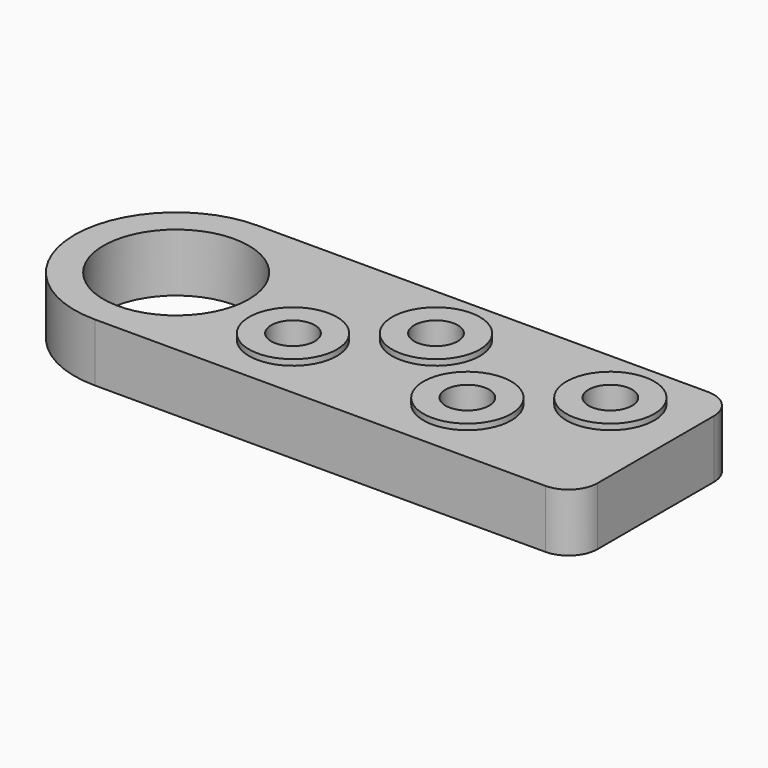
from build123d import *

# Parameters (mm, degrees)
F0_R         = 12.5
F1_DEPTH     = 10
F2_R         = 7.55
F2_R_2       = 3.75
F3_DEPTH     = 1
F4_DEPTH     = 9
F5_TEXT_SIZE = 5.5555555556
F6_DEPTH     = 1


# Not quite as in the source:
# - Text() gives the source's letters only with a copy of the font that has no kerning and outlines rounded to 1/6400 em; it was checked with that copy


with BuildPart() as f1:
    # F0 (on Top) → F1 (new body)
    with BuildSketch(Plane.XY):
        with BuildLine():
            ThreePointArc((0, 17.5), (5.1256313292, 5.1256313292), (17.5, 0))
            Line((17.5, 0), (95, 0))
            ThreePointArc((95, 0), (98.5355339059, 1.4644660941), (100, 5))
            Line((100, 5), (100, 30))
            ThreePointArc((100, 30), (98.5355339059, 33.5355339059), (95, 35))
            Line((95, 35), (17.5, 35))
            ThreePointArc((17.5, 35), (5.1256313292, 29.8743686708), (0, 17.5))
        make_face()
        with Locations((17.5, 17.5)):
            Circle(F0_R, mode=Mode.SUBTRACT)
    extrude(amount=F1_DEPTH)

    # F2 (on face) → F3 (join)
    with BuildSketch(Plane.XY.offset(10)):
        with Locations((42, 12)):
            Circle(F2_R)
        with Locations((42, 12)):
            Circle(F2_R_2, mode=Mode.SUBTRACT)
        with Locations((57, 24)):
            Circle(F2_R)
        with Locations((57, 24)):
            Circle(F2_R_2, mode=Mode.SUBTRACT)
        with Locations((72, 12)):
            Circle(F2_R)
        with Locations((72, 12)):
            Circle(F2_R_2, mode=Mode.SUBTRACT)
        with Locations((87, 24)):
            Circle(F2_R)
        with Locations((87, 24)):
            Circle(F2_R_2, mode=Mode.SUBTRACT)
    extrude(amount=F3_DEPTH)

    # F4 (cut): faces of the model
    f4_faces = [f1.faces().sort_by_distance(p)[0] for p in [
        (42, 12, 10),
        (57, 24, 10),
        (72, 12, 10),
        (87, 24, 10),
    ]]
    extrude(f4_faces, amount=-F4_DEPTH, mode=Mode.SUBTRACT)

    # F5 (on face) → F6 (cut)
    with BuildSketch(Plane(origin=(0, 0, 0), x_dir=(1, 0, 0), z_dir=(0, 0, -1))):
        with Locations((30, -9)):
            Text('962, 1008', F5_TEXT_SIZE, font='Open Sans', text_align=(TextAlign.LEFT, TextAlign.BOTTOM))
    extrude(amount=-F6_DEPTH, mode=Mode.SUBTRACT)


solid = f1.part
